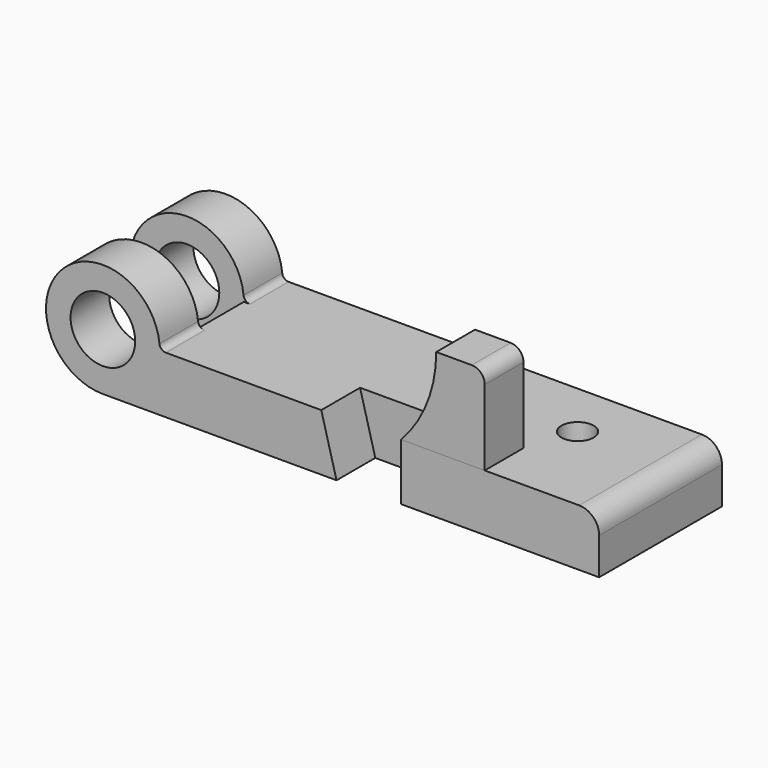
from build123d import *

# Parameters (mm, degrees)
F0_R     = 12.7
F1_DEPTH = 60.325
F2_DEPTH = 19.05
F4_DEPTH = 19.05
F5_W     = 85.049899257
F5_H     = 22.3266
F5_R     = 6.35
F6_DEPTH = 29.464
F7_R     = 7.874
F8_R     = 5.08
F9_R     = 2.54


with BuildPart() as f1:
    # F0 (on Front) → F1 (new body)
    with BuildSketch(Plane.XZ):
        with BuildLine():
            Line((-77.8256, 0), (-172.72, 0))
            ThreePointArc((-172.72, 0), (-210.8772507731, 15.8052507731), (-195.072, -22.352))
            Line((-195.072, -22.352), (0, -22.352))
            Line((0, -22.352), (0, 0))
            Line((0, 0), (-44.9834, 0))
            Line((-44.9834, 0), (-77.8256, 0))
        make_face()
        with Locations((-195.072, 0)):
            Circle(F0_R, mode=Mode.SUBTRACT)
    extrude(amount=-F1_DEPTH)

    # F3 (on face) → F4 (cut)
    with BuildSketch(Plane.XZ):
        Polygon((-77.8256, -22.352), (-77.8256, 0), (-109.22, 0), (-103.2256, -22.352), align=None)
    extrude(amount=-F4_DEPTH, mode=Mode.SUBTRACT)

    # F5 (on face) → F6 (cut, symmetric)
    with BuildSketch(Plane.XY):
        with Locations((-215.2449496285, 30.1625)):
            Rectangle(F5_W, F5_H)
        with Locations((-38.862, 37.973)):
            Circle(F5_R)
    extrude(amount=F6_DEPTH, both=True, mode=Mode.SUBTRACT)

    # F7
    f7_edges = [f1.edges().sort_by_distance(p)[0] for p in [
        (0, 30.1625, 0),
    ]]
    fillet(f7_edges, radius=F7_R)

    # F9
    f9_edges = [f1.edges().sort_by_distance(p)[0] for p in [
        (-172.72, 50.8254, 0),
        (-172.72, 9.4996, 0),
    ]]
    fillet(f9_edges, radius=F9_R)


with BuildPart() as f2:
    # F0 (on Front) → F2 (new body)
    with BuildSketch(Plane.XZ):
        with BuildLine():
            ThreePointArc((-64.0334, 34.798), (-67.6075846384, 16.0823576341), (-77.8256, 0))
            Line((-77.8256, 0), (-44.9834, 0))
            Line((-44.9834, 0), (-44.9834, 34.798))
            Line((-44.9834, 34.798), (-64.0334, 34.798))
        make_face()
    extrude(amount=-F2_DEPTH)

    # F8
    f8_edges = [f2.edges().sort_by_distance(p)[0] for p in [
        (-44.9834, 9.525, 34.798),
    ]]
    fillet(f8_edges, radius=F8_R)


solid = Compound([f1.part, f2.part])
